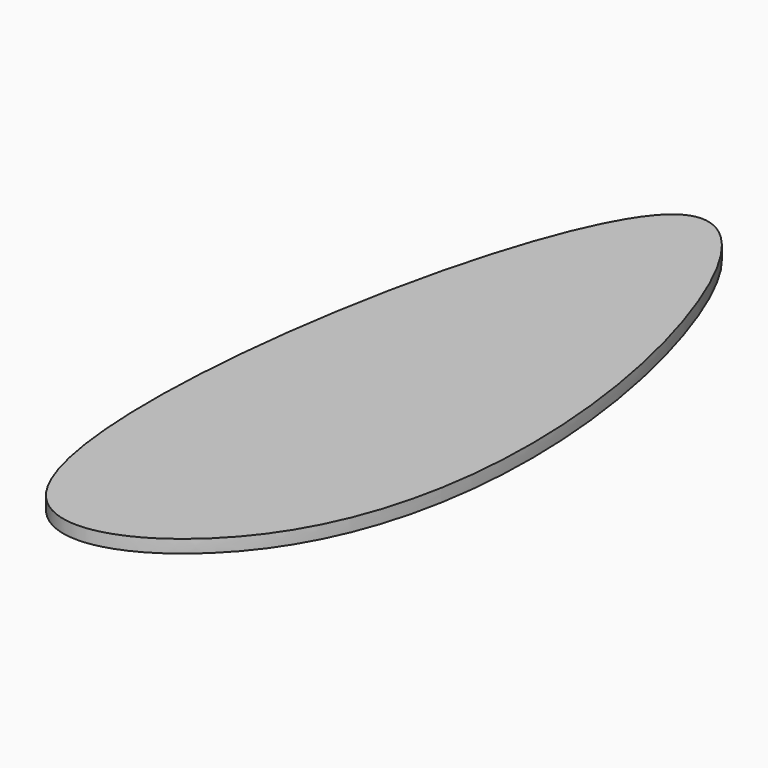
from build123d import *

# Parameters (mm, degrees)
F1_DEPTH = 1.524


with BuildPart() as f1:
    # F0 (on Top) → F1 (new body)
    with BuildSketch(Plane.XY):
        with BuildLine():
            add(Edge.make_bspline(
                [(0, 0), (5.064578753, -7.2696486377), (32.262799099, 6.5531268908), (29.2369527472, 60.2004015822), (5.3085155602, 100.0415820975), (-9.4201512984, 13.5215964432), (0, 0)],
                knots=[0, 0, 0, 0, 0.1861763284, 0.4773380425, 0.6537107492, 1, 1, 1, 1], degree=3))
        make_face()
    extrude(amount=-F1_DEPTH)


solid = f1.part
